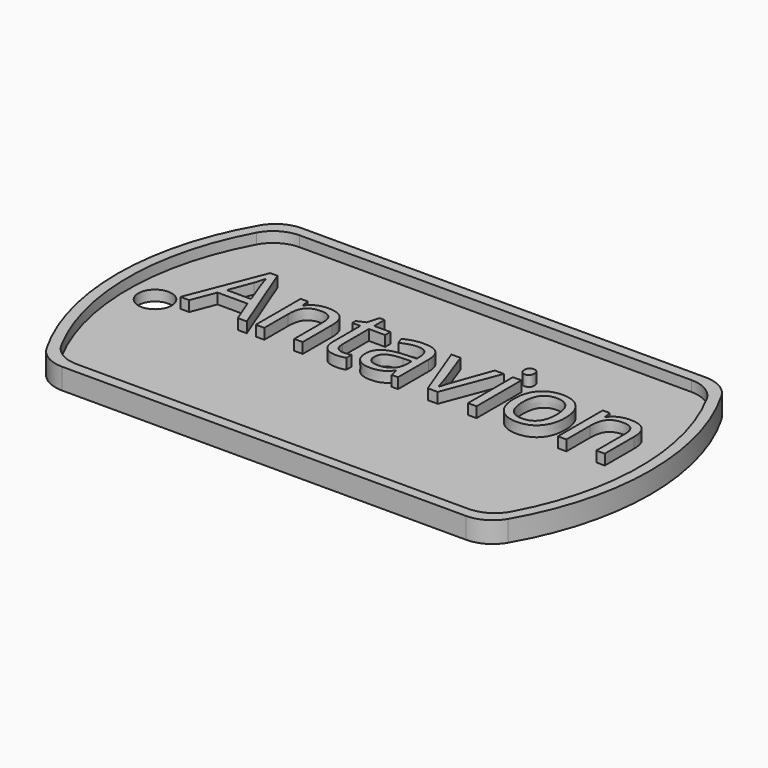
from build123d import *

# Parameters (mm, degrees)
F1_DEPTH     = 1
F3_DEPTH     = 1
F4_R         = 1.5875
F5_DEPTH     = 1
F6_TEXT_SIZE = 9.9928202366
F7_DEPTH     = 1


# Not quite as in the source:
# - Text() gives the source's letters only with a copy of the font that has no kerning and outlines rounded to 1/6400 em; it was checked with that copy


with BuildPart() as f1:
    # F0 (on Top) → F1 (new body)
    with BuildSketch(Plane.XY):
        with BuildLine():
            ThreePointArc((-19.2474145991, 14.2875), (-20.8349145991, 13.862130657), (-21.9970452561, 12.7))
            ThreePointArc((-21.9970452561, 12.7), (-25.4, 0), (-21.9970452561, -12.7))
            ThreePointArc((-21.9970452561, -12.7), (-20.8349145991, -13.862130657), (-19.2474145991, -14.2875))
            Line((-19.2474145991, -14.2875), (19.2474145991, -14.2875))
            ThreePointArc((19.2474145991, -14.2875), (20.8349145991, -13.862130657), (21.9970452561, -12.7))
            ThreePointArc((21.9970452561, -12.7), (25.4, 0), (21.9970452561, 12.7))
            ThreePointArc((21.9970452561, 12.7), (20.8349145991, 13.862130657), (19.2474145991, 14.2875))
            Line((19.2474145991, 14.2875), (-19.2474145991, 14.2875))
        make_face()
    extrude(amount=F1_DEPTH)

    # F2 (on face) → F3 (join)
    with BuildSketch(Plane.XY.offset(1)):
        with BuildLine():
            Line((19.2474145991, 14.2875), (-19.2474145991, 14.2875))
            ThreePointArc((-19.2474145991, 14.2875), (-20.8349145991, 13.862130657), (-21.9970452561, 12.7))
            ThreePointArc((-21.9970452561, 12.7), (-25.4, 0), (-21.9970452561, -12.7))
            ThreePointArc((-21.9970452561, -12.7), (-20.8349145991, -13.862130657), (-19.2474145991, -14.2875))
            Line((-19.2474145991, -14.2875), (19.2474145991, -14.2875))
            ThreePointArc((19.2474145991, -14.2875), (20.8349145991, -13.862130657), (21.9970452561, -12.7))
            ThreePointArc((21.9970452561, -12.7), (25.4, 0), (21.9970452561, 12.7))
            ThreePointArc((21.9970452561, 12.7), (20.8349145991, 13.862130657), (19.2474145991, 14.2875))
        make_face()
        with BuildLine():
            ThreePointArc((-21.4526124879, 11.6252061249), (-20.2856017842, 12.8404540819), (-18.6611352482, 13.2875))
            Line((-18.6611352482, 13.2875), (18.6611352482, 13.2875))
            ThreePointArc((18.6611352482, 13.2875), (20.2856017842, 12.8404540819), (21.4526124879, 11.6252061249))
            ThreePointArc((21.4526124879, 11.6252061249), (24.4, 0), (21.4526124879, -11.6252061249))
            ThreePointArc((21.4526124879, -11.6252061249), (20.2856017842, -12.8404540819), (18.6611352482, -13.2875))
            Line((18.6611352482, -13.2875), (-18.6611352482, -13.2875))
            ThreePointArc((-18.6611352482, -13.2875), (-20.2856017842, -12.8404540819), (-21.4526124879, -11.6252061249))
            ThreePointArc((-21.4526124879, -11.6252061249), (-24.4, 0), (-21.4526124879, 11.6252061249))
        make_face(mode=Mode.SUBTRACT)
    extrude(amount=F3_DEPTH)

    # F4 (on face) → F5 (cut)
    with BuildSketch(Plane.XY.offset(1)):
        with Locations((-21.821282804, 0)):
            Circle(F4_R)
    extrude(amount=-F5_DEPTH, mode=Mode.SUBTRACT)

    # F6 (on face) → F7 (join)
    with BuildSketch(Plane.XY.offset(1)):
        with Locations((-19.3996429443, 0)):
            Text('Antavion', F6_TEXT_SIZE, font='Open Sans', text_align=(TextAlign.LEFT, TextAlign.BOTTOM))
    extrude(amount=F7_DEPTH)


solid = f1.part
